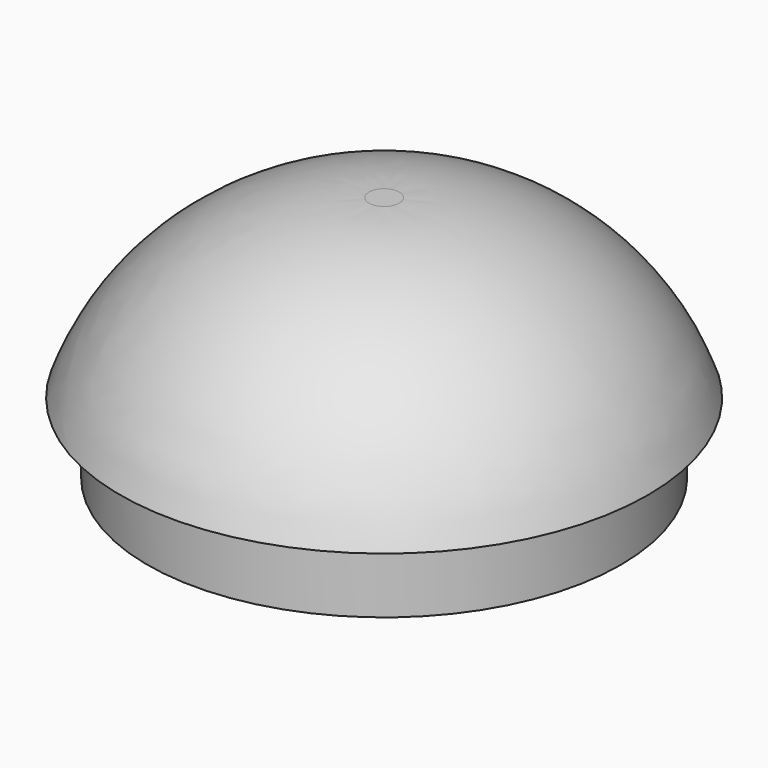
from build123d import *

# Parameters (mm, degrees)
F0_R     = 15
F1_DEPTH = 10
F3_R     = 13.4495
F4_DEPTH = 4
F5_W     = 6
F5_H     = 6
F6_DEPTH = 3
F7_R     = 1.75
F8_DEPTH = 1.5


# Not quite as in the source:
# - a fillet or chamfer that OpenCascade refuses, or shapes differently, is made with other operations: its cross-section is extruded or revolved along the edge and cut away or added


with BuildPart() as f1:
    # F0 (on Top) → F1 (new body)
    with BuildSketch(Plane.XY):
        Circle(F0_R)
    extrude(amount=F1_DEPTH)

    # F2: fillet of radius 15 on 1 edges, made by hand

    # F2_s1 → F2_t2 (revolve, cut)
    with BuildSketch(Plane.XZ):
        with BuildLine():
            ThreePointArc((15, 0), (9.5181184141, 7.2474487139), (0.8578643763, 10))
            Line((0.8578643763, 10), (15, 10))
            Line((15, 10), (15, 0))
        make_face()
    revolve(axis=Axis((0, 0, 10), (0, 0, 1)), mode=Mode.SUBTRACT)

    # F3 (on face) → F4 (join)
    with BuildSketch(Plane(origin=(0, 0, 0), x_dir=(1, 0, 0), z_dir=(0, 0, -1))):
        Circle(F3_R)
    extrude(amount=F4_DEPTH)

    # F5 (on face) → F6 (cut)
    with BuildSketch(Plane(origin=(0, 0, -4), x_dir=(1, 0, 0), z_dir=(0, 0, -1))):
        Rectangle(F5_W, F5_H)
    extrude(amount=-F6_DEPTH, mode=Mode.SUBTRACT)

    # F7 (on face) → F8 (cut)
    with BuildSketch(Plane(origin=(0, 0, -1), x_dir=(1, 0, 0), z_dir=(0, 0, -1))):
        Circle(F7_R)
    extrude(amount=-F8_DEPTH, mode=Mode.SUBTRACT)


solid = f1.part
